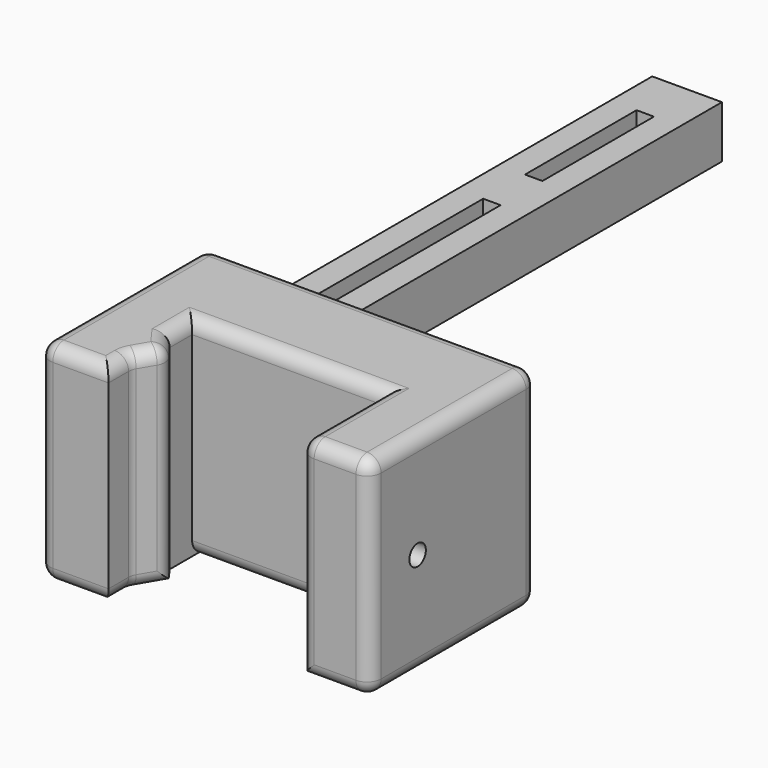
from build123d import *

# Parameters (mm, degrees)
F0_W      = 120.65
F0_H      = 76.2
F2_DEPTH  = 38.1
F1_W      = 69.85
F1_H      = 101.6
F3_DEPTH  = 38.1
F4_R      = 3.7467551061
F5_DEPTH  = 38.1
F6_W      = 25.4
F6_H      = 19.05
F7_DEPTH  = 203.2
F8_W      = 6.35
F8_H      = 50.8
F8_H_2    = 76.2
F9_DEPTH  = 47.626
F11_DEPTH = 38.1
F12_R     = 5.08


with BuildPart() as f2:
    # F0 (on Top) → F2 (new body, symmetric)
    with BuildSketch(Plane.XY):
        Rectangle(F0_W, F0_H)
    extrude(amount=F2_DEPTH, both=True)

    # F1 (on face) → F3 (cut, symmetric)
    with BuildSketch(Plane.XY):
        with Locations((0, -50.8)):
            Rectangle(F1_W, F1_H)
    extrude(amount=F3_DEPTH, both=True, mode=Mode.SUBTRACT)

    # F4 (on face) → F5 (cut, symmetric)
    with BuildSketch(Plane.YZ.offset(60.325)):
        with Locations((-16.3753926754, 0)):
            Circle(F4_R)
    extrude(amount=F5_DEPTH, both=True, mode=Mode.SUBTRACT)

    # F6 (on face) → F7 (join)
    with BuildSketch(Plane(origin=(0, 38.1, 0), x_dir=(-1, 0, 0), z_dir=(0, 1, 0))):
        with Locations((47.625, 0)):
            Rectangle(F6_W, F6_H)
    extrude(amount=F7_DEPTH)

    # F8 (on face) → F9 (cut, through all)
    with BuildSketch(Plane.XY.offset(9.525)):
        with Locations((-47.625, 196.85)):
            Rectangle(F8_W, F8_H)
        with Locations((-47.625, 114.3)):
            Rectangle(F8_W, F8_H_2)
    extrude(amount=-F9_DEPTH, mode=Mode.SUBTRACT)

    # F10 (on Top) → F11 (join, symmetric)
    with BuildSketch(Plane.XY):
        Polygon((-29.2977448553, -18.0150475353), (-34.9880978465, -10.1638017222), (-35.0601263344, -27.8110988438), align=None)
    extrude(amount=F11_DEPTH, both=True)

    # F12
    f12_edges = [f2.edges().sort_by_distance(p)[0] for p in [
        (60.325, -38.1, 0),
        (60.325, 0, 38.1),
        (60.325, 38.1, 0),
        (60.325, 0, -38.1),
        (0, 38.1, 38.1),
        (-60.325, 38.1, 23.8125),
        (-60.325, 38.1, -23.8125),
        (0, 38.1, -38.1),
        (-60.325, 0, 38.1),
        (-60.325, -38.1, 0),
        (-60.325, 0, -38.1),
        (34.925, -38.1, 0),
        (-34.925, -27.581384, 0),
        (-32.111372, -22.798216, 38.1),
        (-29.297745, -18.015048, 0),
        (-32.111372, -22.798216, -38.1),
        (0, 0, 38.1),
        (0, 0, -38.1),
        (47.625, -38.1, 38.1),
        (47.625, -38.1, -38.1),
        (-47.625, -38.1, 38.1),
        (-47.625, -38.1, -38.1),
        (-34.925, -5.12543, 38.1),
        (-32.111372, -14.132954, 38.1),
        (-34.925, -32.840692, 38.1),
        (34.925, -19.05, 38.1),
        (-34.925, -32.840692, -38.1),
    ]]
    fillet(f12_edges, radius=F12_R)


solid = f2.part
